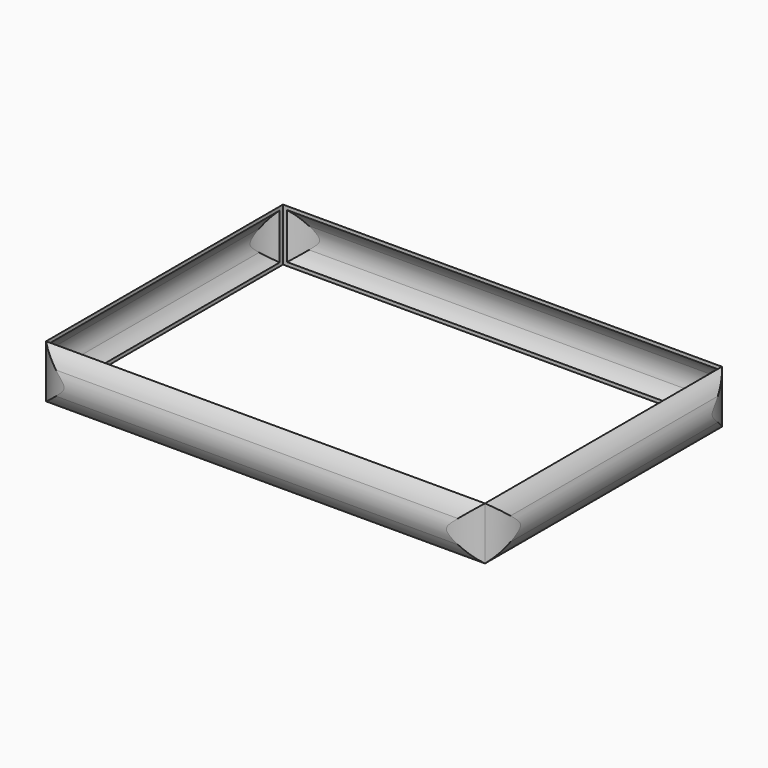
from build123d import *

# Parameters (mm, degrees)
F3_W          = 83
F3_H          = 10
F5_DEPTH      = 2.5
F4_W          = 56
F4_H          = 10
F6_DEPTH      = 2.5
F7_T1_DEPTH   = 42.4807635378
F7_2_T1_DEPTH = 42.4807635378
F8_T1_DEPTH   = 96.8172078217
F8_2_T1_DEPTH = 69.8172078217
F9_R          = 6
F9_2_R        = 6
F10_T         = -0.5
F10_2_T       = -0.5


# Not quite as in the source:
# - a fillet or chamfer that OpenCascade refuses, or shapes differently, is made with other operations: its cross-section is extruded or revolved along the edge and cut away or added
# - a feature of the source that left no trace in its solid (it failed there, or was rolled back) is left out
# - the program builds the solid bodies; features that only make, move or delete a surface that nothing else refers to are left out


with BuildPart() as f5:
    # F3 (on Front) → F5 (new body)
    with BuildSketch(Plane.XZ):
        Rectangle(F3_W, F3_H)
    extrude(amount=F5_DEPTH)

    # F7: fillet of radius 9.69 on 2 edges, made by hand

    # F7_s2 → F7_t1 (cut)
    with BuildSketch(Plane.XY.offset(-21.2403817689)):
        with BuildLine():
            ThreePointArc((-41.5, 0), (-38.4841490035, -1.8534285534), (-35.0038472924, -2.5))
            Line((-35.0038472924, -2.5), (-35.0038472924, -2.6938))
            Line((-35.0038472924, -2.6938), (-41.5, -2.6938))
            Line((-41.5, -2.6938), (-41.6938, -2.5))
            ThreePointArc((-41.6938, -2.5), (-41.6938, -1.25), (-41.6299230542, -0.1438))
            Line((-41.6299230542, -0.1438), (-41.5, 0))
        make_face()
        with BuildLine():
            ThreePointArc((41.5, 0), (38.4841490035, -1.8534285534), (35.0038472924, -2.5))
            Line((35.0038472924, -2.5), (35.0038472924, -2.6938))
            Line((35.0038472924, -2.6938), (41.5, -2.6938))
            Line((41.5, -2.6938), (41.6938, -2.5))
            ThreePointArc((41.6938, -2.5), (41.6938, -1.25), (41.6299230542, -0.1438))
            Line((41.6299230542, -0.1438), (41.5, 0))
        make_face()
    extrude(amount=F7_T1_DEPTH, mode=Mode.SUBTRACT)

    # F8: fillet of radius 7 on 2 edges, made by hand

    # F8_s2 → F8_t1 (cut)
    with BuildSketch(Plane.YZ.offset(-48.4086039109)):
        with BuildLine():
            ThreePointArc((0, 5), (-1.8442887702, 2.5961372442), (-2.5, -0.3619026474))
            Line((-2.5, -0.3619026474), (-2.5, 5))
            Line((-2.5, 5), (0, 5))
        make_face()
        with BuildLine():
            ThreePointArc((0, -5), (-1.8442887702, -2.5961372442), (-2.5, 0.3619026474))
            Line((-2.5, 0.3619026474), (-2.5, -5))
            Line((-2.5, -5), (0, -5))
        make_face()
    extrude(amount=F8_T1_DEPTH, mode=Mode.SUBTRACT)

    # F9
    f9_edges = [f5.edges().sort_by_distance(p)[0] for p in [
        (0, -2.490638, 0),
    ]]
    fillet(f9_edges, radius=F9_R)

    # F10
    f10_openings = [f5.faces().sort_by_distance(p)[0] for p in [
        (0, 0, 0),
    ]]
    offset(amount=F10_T, openings=f10_openings)


with BuildPart() as f6:
    # F4 (on offset) → F6 (new body)
    with BuildSketch(Plane.YZ.offset(41.5)):
        with Locations((28, -0.0004571676)):
            Rectangle(F4_W, F4_H)
    extrude(amount=F6_DEPTH)

    # F7#2: fillet of radius 9.69 on 2 edges, made by hand

    # F7_2_s2 → F7_2_t1 (cut)
    with BuildSketch(Plane.XY.offset(-21.2408389365)):
        with BuildLine():
            ThreePointArc((41.5, 0), (43.3534285534, 3.0158509965), (44, 6.4961527076))
            Line((44, 6.4961527076), (44.1938, 6.4961527076))
            Line((44.1938, 6.4961527076), (44.1938, 0))
            Line((44.1938, 0), (44, -0.1938))
            ThreePointArc((44, -0.1938), (42.75, -0.1938), (41.6438, -0.1299230542))
            Line((41.6438, -0.1299230542), (41.5, 0))
        make_face()
        with BuildLine():
            ThreePointArc((41.5, 56), (43.3534285534, 52.9841490035), (44, 49.5038472924))
            Line((44, 49.5038472924), (44.1938, 49.5038472924))
            Line((44.1938, 49.5038472924), (44.1938, 56))
            Line((44.1938, 56), (44, 56.1938))
            ThreePointArc((44, 56.1938), (42.75, 56.1938), (41.6438, 56.1299230542))
            Line((41.6438, 56.1299230542), (41.5, 56))
        make_face()
    extrude(amount=F7_2_T1_DEPTH, mode=Mode.SUBTRACT)

    # F8#2: fillet of radius 7 on 2 edges, made by hand

    # F8_2_s2 → F8_2_t1 (cut)
    with BuildSketch(Plane.XZ.offset(-62.9086039109)):
        with BuildLine():
            ThreePointArc((41.5, 4.9995428324), (43.3442887702, 2.5956800765), (44, -0.362359815))
            Line((44, -0.362359815), (44, 4.9995428324))
            Line((44, 4.9995428324), (41.5, 4.9995428324))
        make_face()
        with BuildLine():
            ThreePointArc((41.5, -5.0004571676), (43.3442887702, -2.5965944118), (44, 0.3614454798))
            Line((44, 0.3614454798), (44, -5.0004571676))
            Line((44, -5.0004571676), (41.5, -5.0004571676))
        make_face()
    extrude(amount=F8_2_T1_DEPTH, mode=Mode.SUBTRACT)

    # F9#2
    f9_2_edges = [f6.edges().sort_by_distance(p)[0] for p in [
        (43.990638, 28, -0.000457),
    ]]
    fillet(f9_2_edges, radius=F9_2_R)

    # F10#2
    f10_2_openings = [f6.faces().sort_by_distance(p)[0] for p in [
        (41.5, 28, -0.000457),
    ]]
    offset(amount=F10_2_T, openings=f10_2_openings)


with BuildPart() as f11_1:
    # F11: instance of F6
    add(f6.part.mirror(Plane.YZ))


with BuildPart() as f12_1:
    # F12: instance of F5
    add(f5.part.mirror(Plane.XZ))


with BuildPart() as f12_1_1:
    # F13: moved
    add(f12_1.part.moved(Location((0, 56, 0))))


solid = Compound([f5.part, f6.part, f11_1.part, f12_1_1.part])
